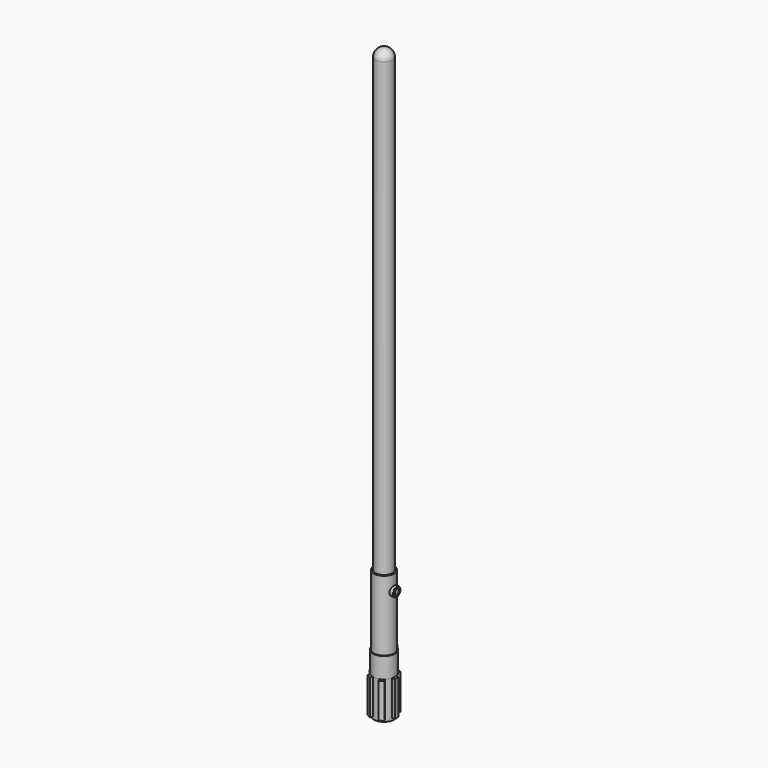
from build123d import *

# Parameters (mm, degrees)
F2_R      = 22.225
F3_DEPTH  = 139.7
F4_W      = 10.16
F4_H      = 76.2
F7_COUNT  = 6
F8_R      = 22.225
F9_DEPTH  = 44.45
F10_R     = 10.16
F10_R_2   = 6.35
F11_REACH = 84.6178195874
F12_SIZE  = 2.54
F13_R     = 0.762
F14_R     = 5.715
F15_REACH = 72.0454610179
F16_R     = 0.508
F17_R     = 18.669
F18_DEPTH = 1000
F19_R     = 18.288


with BuildPart() as f3:
    # F2 (on Top) → F3 (new body, symmetric)
    with BuildSketch(Plane.XY):
        Circle(F2_R)
    extrude(amount=F3_DEPTH, both=True)


with BuildPart() as f5:
    # F4 (on offset) → F5 (new body, up to the next surface of F3)
    with BuildSketch(Plane.YZ.offset(27.94)):
        with Locations((0, -96.52)):
            Rectangle(F4_W, F4_H)
    extrude(until=Until.NEXT, target=f3.part, dir=(-1, 0, 0))


with BuildPart() as f7_1:
    # F7: instance of F5
    add(f5.part.rotate(Axis((0, 0, 26.7843), (0, 0, -1)), 1 * 360 / F7_COUNT))


with BuildPart() as f7_2:
    # F7: instance of F5
    add(f5.part.rotate(Axis((0, 0, 26.7843), (0, 0, -1)), 2 * 360 / F7_COUNT))


with BuildPart() as f7_3:
    # F7: instance of F5
    add(f5.part.rotate(Axis((0, 0, 26.7843), (0, 0, -1)), 3 * 360 / F7_COUNT))


with BuildPart() as f7_4:
    # F7: instance of F5
    add(f5.part.rotate(Axis((0, 0, 26.7843), (0, 0, -1)), 4 * 360 / F7_COUNT))


with BuildPart() as f7_5:
    # F7: instance of F5
    add(f5.part.rotate(Axis((0, 0, 26.7843), (0, 0, -1)), 5 * 360 / F7_COUNT))


with BuildPart() as f9:
    # F8 (on offset) → F9 (new body)
    with BuildSketch(Plane.XY.offset(-12.7)):
        with BuildLine():
            Line((-6.35, 28.3594845304), (-6.35, 23.2794845304))
            ThreePointArc((-6.35, 23.2794845304), (0, -24.13), (6.35, 23.2794845304))
            Line((6.35, 23.2794845304), (6.35, 28.3594845304))
            Line((6.35, 28.3594845304), (-6.35, 28.3594845304))
        make_face()
        Circle(F8_R, mode=Mode.SUBTRACT)
    extrude(amount=-F9_DEPTH)


with BuildPart() as f11:
    f11_end = f3.part.faces().sort_by_distance((-22.225, 0, 0))[0]
    # F10 (on offset) → F11 (new body, up to a face of F3 that its end follows)
    with BuildSketch(Plane.YZ.offset(27.94)):
        with Locations((0, 106.68)):
            Circle(F10_R)
        with Locations((0, 106.68)):
            Circle(F10_R_2, mode=Mode.SUBTRACT)
    f11_long = extrude(amount=-F11_REACH, mode=Mode.PRIVATE)
    add(split(f11_long, bisect_by=f11_end, keep=Keep.ALL, mode=Mode.PRIVATE).solids().sort_by_distance((27.94, -9.8726318041, 106.68))[0])

    # F12
    f12_edges = [f11.edges().sort_by_distance(p)[0] for p in [
        (27.94, -6.35, 106.68),
    ]]
    chamfer(f12_edges, length=F12_SIZE)

    # F13
    f13_edges = [f11.edges().sort_by_distance(p)[0] for p in [
        (26.67, 7.62, 106.68),
        (27.94, -8.89, 106.68),
        (25.4, -6.35, 106.68),
        (27.94, -10.16, 106.68),
    ]]
    fillet(f13_edges, radius=F13_R)


with BuildPart() as f15:
    f15_end = f3.part.faces().sort_by_distance((-22.225, 0, 0))[0]
    # F14 (on offset) → F15 (new body, up to a face of F3 that its end follows)
    with BuildSketch(Plane.YZ.offset(27.94)):
        with Locations((0, 106.68)):
            Circle(F14_R)
    f15_long = extrude(amount=-F15_REACH, mode=Mode.PRIVATE)
    add(split(f15_long, bisect_by=f15_end, keep=Keep.ALL, mode=Mode.PRIVATE).solids().sort_by_distance((27.94, 0, 106.68))[0])

    # F16
    f16_edges = [f15.edges().sort_by_distance(p)[0] for p in [
        (27.94, -5.715, 106.68),
    ]]
    fillet(f16_edges, radius=F16_R)


with BuildPart() as f18:
    # F17 (on face) → F18 (new body)
    with BuildSketch(Plane.XY.offset(139.7)):
        Circle(F17_R)
    extrude(amount=F18_DEPTH)

    # F19
    f19_edges = [f18.edges().sort_by_distance(p)[0] for p in [
        (-18.669, 0, 1139.7),
    ]]
    fillet(f19_edges, radius=F19_R)


solid = Compound([f3.part, f5.part, f7_1.part, f7_2.part, f7_3.part, f7_4.part, f7_5.part, f9.part, f11.part, f15.part, f18.part])
